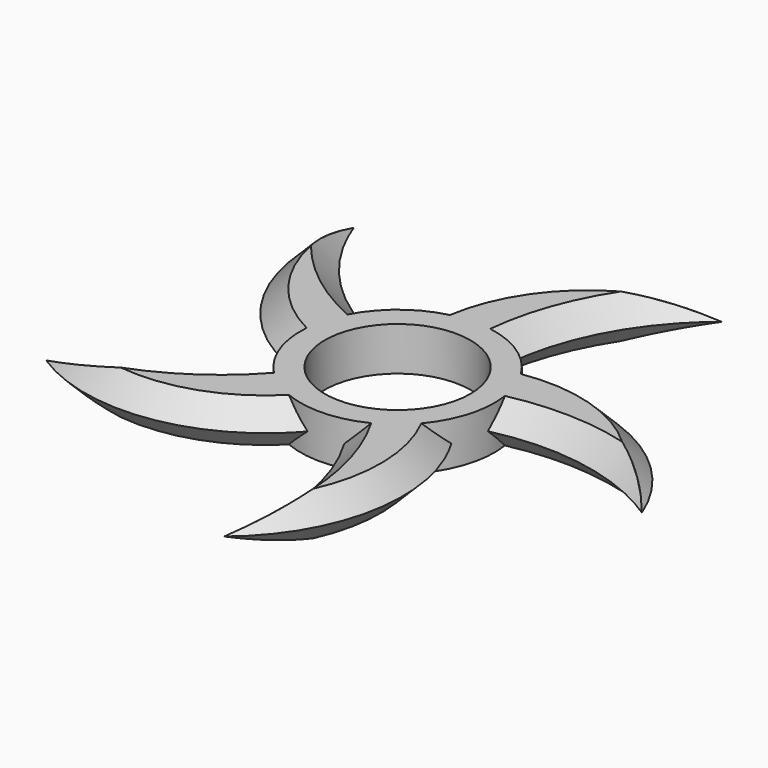
from build123d import *

# Parameters (mm, degrees)
F0_R        = 20
F0_R_2      = 15
F1_DEPTH    = 9
F3_DEPTH    = 9
F4_SIZE     = 5
F5_T2_ANGLE = 123.748279
F5_T4_ANGLE = 80.142153
F6_COUNT    = 5


# Not quite as in the source:
# - a fillet or chamfer that OpenCascade refuses, or shapes differently, is made with other operations: its cross-section is extruded or revolved along the edge and cut away or added


with BuildPart() as f1:
    # F0 (on Top) → F1 (new body)
    with BuildSketch(Plane.XY):
        Circle(F0_R)
        Circle(F0_R_2, mode=Mode.SUBTRACT)
    extrude(amount=F1_DEPTH)

    # F2 (on face) → F3 (join)
    with BuildSketch(Plane(origin=(0, 0, 0), x_dir=(1, 0, 0), z_dir=(0, 0, -1))):
        with BuildLine():
            ThreePointArc((-10.012645, -17.313201), (1.770458, -41.944997), (27.075166, -52.203585))
            ThreePointArc((27.075166, -52.203585), (13.969746, -37.260438), (8.208542, -18.237868))
            ThreePointArc((8.208542, -18.237868), (-1.013632, -19.974297), (-10.012645, -17.313201))
        make_face()
    extrude(amount=-F3_DEPTH)

    # F4
    f4_edges = [f1.edges().sort_by_distance(p)[0] for p in [
        (13.969746, 37.260438, 9),
        (1.770458, 41.944997, 9),
    ]]
    chamfer(f4_edges, length=F4_SIZE)

    # F5: chamfer of 5 on 2 edges, made by hand

    # F5_s1 → F5_t2 (revolve, cut)
    with BuildSketch(Plane(origin=(-1.7509, 6.477661, 0), x_dir=(0, 0, 1), z_dir=(0.260934, -0.965357, 0))):
        Polygon((5, 7.316767), (0, 2.316767), (0, 7.316767), align=None)
    revolve(axis=Axis((27.658151, 14.426873, 0), (0, 0, -1)), revolution_arc=F5_T2_ANGLE, mode=Mode.SUBTRACT)

    # F5_s3 → F5_t4 (revolve, cut)
    with BuildSketch(Plane(origin=(52.885681, 20.17231, 0), x_dir=(0, 0, 1), z_dir=(0.934338, 0.356387, 0))):
        Polygon((0, -45.874117), (5, -40.874117), (0, -40.874117), align=None)
    revolve(axis=Axis((55.077177, 14.426873, 0), (0, 0, 1)), revolution_arc=F5_T4_ANGLE, mode=Mode.SUBTRACT)

    # F6: F1 ×5 about axis
    f6_axis = Axis((0, 0, 0), (0, 0, -1))


with BuildPart() as f1_1:
    add(f1.part)
    for i in range(1, F6_COUNT):
        add(f1.part.rotate(f6_axis, i * 360 / F6_COUNT))


solid = f1_1.part
